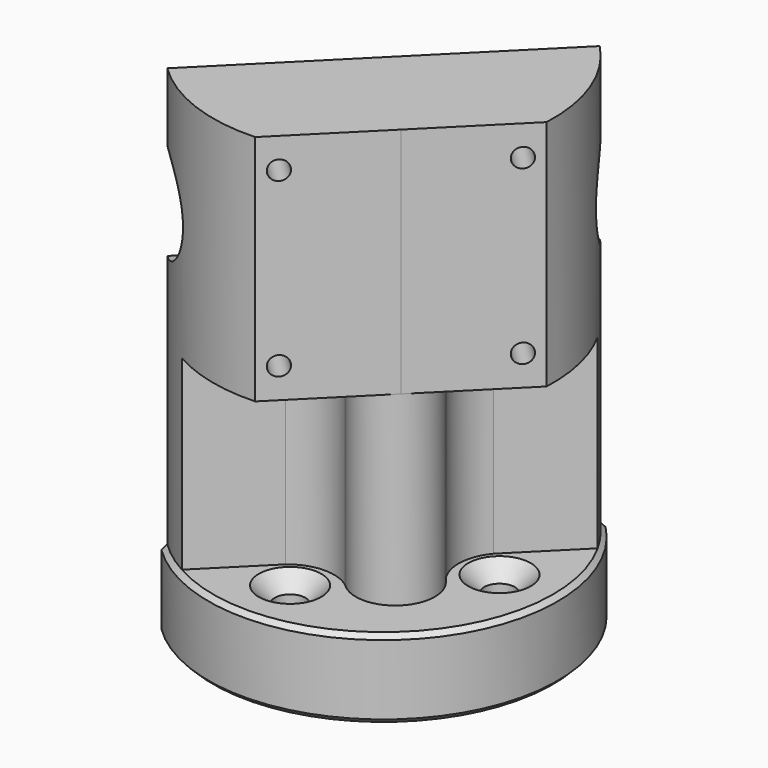
from build123d import *

# Parameters (mm, degrees)
F1_ANGLE_BACK  = 45
F1_ANGLE       = 180
F2_SIZE        = 1
F4_D           = 6.6
F4_CSINK_D     = 13.44
F4_CSINK_ANGLE = 90
F6_DEPTH       = 40
F8_DEPTH       = 50
F12_D          = 4.1
F13_W          = 100.6186008453
F13_H          = 151.657152921
F14_DEPTH      = 0.5


# Not quite as in the source:
# - a feature names something its author has since deleted; it is built from what else it names


with BuildPart() as f1:
    # F0 (on Front) → F1 (revolve)
    with BuildSketch(Plane.XZ, mode=Mode.PRIVATE) as f1_sk:
        Polygon((0, 10), (0, 0), (31.6, 0), (31.6, -7), (37.5, -7), (37.5, 10), align=None)
    revolve(f1_sk.sketch.rotate(Axis((0, 0, 5), (0, 0, -1)), -F1_ANGLE_BACK), axis=Axis((0, 0, 5), (0, 0, -1)), revolution_arc=F1_ANGLE)

    # F2
    f2_edges = [f1.edges().sort_by_distance(p)[0] for p in [
        (22.344574, -22.344574, -7),
        (26.516504, -26.516504, -7),
        (26.516504, -26.516504, 10),
    ]]
    chamfer(f2_edges, length=F2_SIZE)

    # F4 (through all)
    with Locations(Plane.XY.offset(10)):
        with Locations((25, 0), (0, -25)):
            CounterSinkHole(F4_D / 2, F4_CSINK_D / 2, counter_sink_angle=F4_CSINK_ANGLE)

    # F5 (on face) → F6 (join)
    with BuildSketch(Plane.XY.offset(10)):
        with BuildLine():
            Line((19.4820004924, 5.3398648686), (7.0710678119, -7.0710678119))
            Line((7.0710678119, -7.0710678119), (-5.3398648686, -19.4820004924))
            ThreePointArc((-5.3398648686, -19.4820004924), (0.79408889, -17.1167209324), (7.0710678119, -19.0710678119))
            ThreePointArc((7.0710678119, -19.0710678119), (19.0710678119, -19.0710678119), (19.0710678119, -7.0710678119))
            ThreePointArc((19.0710678119, -7.0710678119), (17.1167209324, -0.79408889), (19.4820004924, 5.3398648686))
        make_face()
        with BuildLine():
            Line((7.0710678119, -7.0710678119), (0, 0))
            Line((0, 0), (-25.8093975133, -25.8093975133))
            ThreePointArc((-25.8093975133, -25.8093975133), (-21.9914756212, -29.1311688746), (-17.7507975491, -31.8929331729))
            Line((-17.7507975491, -31.8929331729), (-5.3398648686, -19.4820004924))
            Line((-5.3398648686, -19.4820004924), (7.0710678119, -7.0710678119))
        make_face()
        with BuildLine():
            Line((25.8093975133, 25.8093975133), (0, 0))
            Line((0, 0), (7.0710678119, -7.0710678119))
            Line((7.0710678119, -7.0710678119), (19.4820004924, 5.3398648686))
            Line((19.4820004924, 5.3398648686), (31.8929331729, 17.7507975491))
            ThreePointArc((31.8929331729, 17.7507975491), (29.1311688746, 21.9914756212), (25.8093975133, 25.8093975133))
        make_face()
    extrude(amount=F6_DEPTH)

    # F7 (on face) → F8 (join)
    with BuildSketch(Plane.XY.offset(50)):
        with BuildLine():
            ThreePointArc((36.4612769111, -1.6808587126), (35.531279534, 8.3533331479), (31.8929331729, 17.7507975491))
            Line((31.8929331729, 17.7507975491), (19.4820004924, 5.3398648686))
            ThreePointArc((19.4820004924, 5.3398648686), (17.1167209324, -0.79408889), (19.0710678119, -7.0710678119))
            ThreePointArc((19.0710678119, -7.0710678119), (21.5563491861, -13.0710678119), (19.0710678119, -19.0710678119))
            Line((19.0710678119, -19.0710678119), (36.4612769111, -1.6808587126))
        make_face()
        with BuildLine():
            Line((-5.3398648686, -19.4820004924), (-17.7507975491, -31.8929331729))
            ThreePointArc((-17.7507975491, -31.8929331729), (-8.3533331479, -35.531279534), (1.6808587126, -36.4612769111))
            Line((1.6808587126, -36.4612769111), (19.0710678119, -19.0710678119))
            ThreePointArc((19.0710678119, -19.0710678119), (13.0710678119, -21.5563491861), (7.0710678119, -19.0710678119))
            ThreePointArc((7.0710678119, -19.0710678119), (0.79408889, -17.1167209324), (-5.3398648686, -19.4820004924))
        make_face()
        with BuildLine():
            ThreePointArc((31.8929331729, 17.7507975491), (29.1311688746, 21.9914756212), (25.8093975133, 25.8093975133))
            Line((25.8093975133, 25.8093975133), (-25.8093975133, -25.8093975133))
            ThreePointArc((-25.8093975133, -25.8093975133), (-21.9914756212, -29.1311688746), (-17.7507975491, -31.8929331729))
            Line((-17.7507975491, -31.8929331729), (-5.3398648686, -19.4820004924))
            ThreePointArc((-5.3398648686, -19.4820004924), (0.79408889, -17.1167209324), (7.0710678119, -19.0710678119))
            ThreePointArc((7.0710678119, -19.0710678119), (13.0710678119, -21.5563491861), (19.0710678119, -19.0710678119))
            ThreePointArc((19.0710678119, -19.0710678119), (21.5563491861, -13.0710678119), (19.0710678119, -7.0710678119))
            ThreePointArc((19.0710678119, -7.0710678119), (17.1167209324, -0.79408889), (19.4820004924, 5.3398648686))
            Line((19.4820004924, 5.3398648686), (31.8929331729, 17.7507975491))
        make_face()
    extrude(amount=F8_DEPTH)

    # F9 (on face) → F10 (revolve, cut)
    with BuildSketch(Plane(origin=(0, 0, 0), x_dir=(-0.7071067812, -0.7071067812, 0), z_dir=(-0.7071067812, 0.7071067812, 0))):
        Polygon((36.5, 85.5), (-36.5, 86.5), (-36.5, 75), (36.5, 75), align=None)
    revolve(axis=Axis((0, 0, 75), (-0.7071067812, -0.7071067812, 0)), mode=Mode.SUBTRACT)

    # F12 (through all)
    with Locations(Plane(origin=(19.0710678119, -19.0710678119, 0), x_dir=(0.7071067812, 0.7071067812, 0), z_dir=(0.7071067812, -0.7071067812, 0))):
        with Locations((20.5934695606, 93.5), (20.5934695606, 56.5), (-20.5934695606, 56.5), (-20.5934695606, 93.5)):
            Hole(F12_D / 2)

    # F13 (on face) → F14 (cut)
    with BuildSketch(Plane(origin=(0, 0, 0), x_dir=(-0.7071067812, -0.7071067812, 0), z_dir=(-0.7071067812, 0.7071067812, 0))):
        with Locations((-1.9399225712, 37.7359148115)):
            Rectangle(F13_W, F13_H)
    extrude(amount=-F14_DEPTH, mode=Mode.SUBTRACT)


solid = f1.part
